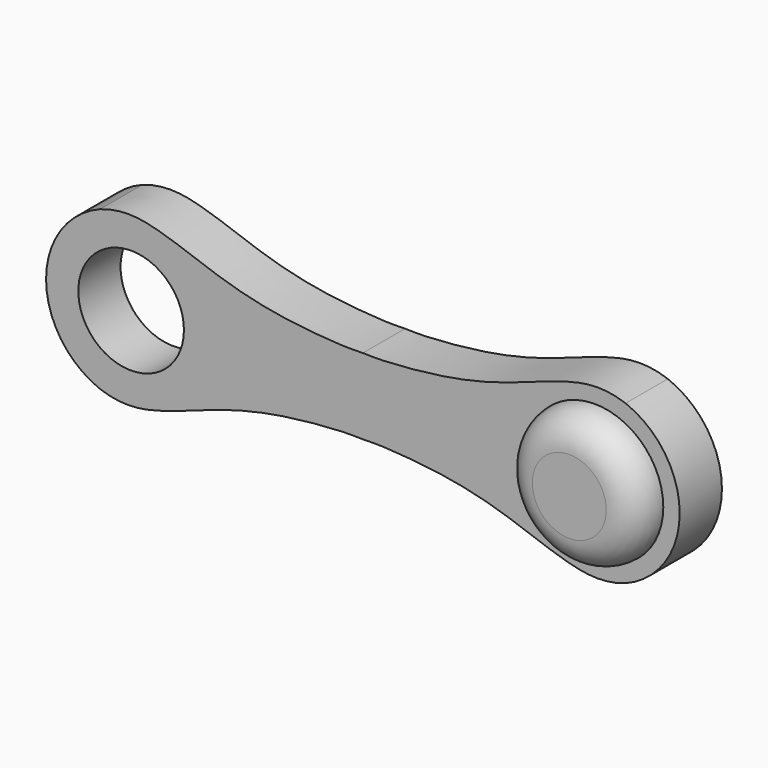
from build123d import *

# Parameters (mm, degrees)
F0_R     = 12.7
F0_R_2   = 16.51
F1_DEPTH = 12.7
F2_DEPTH = 20.32
F3_R     = 7.61999


# Not quite as in the source:
# - a fillet or chamfer is up to 0.001 mm smaller than in the source, because OpenCascade refuses the exact size


with BuildPart() as f1:
    # F0 (on Front) → F1 (new body)
    with BuildSketch(Plane.XZ):
        with BuildLine():
            add(Edge.make_bspline(
                [(63.1930127424, -19.05), (57.8929819167, -20.9148749709), (49.1822585518, -19.6780685204), (34.4123652883, -13.7010865969), (20.7204562035, -10.3509186108), (5.798157397, -8.9775289718), (1.5977957695, -9.0970061045), (0, -9.1456407681)],
                knots=[0, 0, 0, 0, 0.2119684652, 0.4335943825, 0.6511337867, 0.8674060842, 1, 1, 1, 1], degree=3))
            ThreePointArc((63.1930127424, -19.05), (76.2, 0), (63.1930127424, 19.05))
            add(Edge.make_bspline(
                [(63.1930127424, 19.05), (57.8929819167, 20.9148749709), (49.1822585518, 19.6780685204), (34.4123652883, 13.7010865969), (20.7204562035, 10.3509186108), (5.798157397, 8.9775289718), (1.5977957695, 9.0970061045), (0, 9.1456407681)],
                knots=[0, 0, 0, 0, 0.2119684652, 0.4335943825, 0.6511337867, 0.8674060842, 1, 1, 1, 1], degree=3))
            add(Edge.make_bspline(
                [(-63.1930127424, 19.05), (-57.8929819167, 20.9148749709), (-49.1822585518, 19.6780685204), (-34.4123652883, 13.7010865969), (-20.7204562035, 10.3509186108), (-5.798157397, 8.9775289718), (-1.5977957695, 9.0970061045), (0, 9.1456407681)],
                knots=[0, 0, 0, 0, 0.2119684652, 0.4335943825, 0.6511337867, 0.8674060842, 1, 1, 1, 1], degree=3))
            ThreePointArc((-63.1930127424, 19.05), (-76.2, 0), (-63.1930127424, -19.05))
            add(Edge.make_bspline(
                [(-63.1930127424, -19.05), (-57.8929819167, -20.9148749709), (-49.1822585518, -19.6780685204), (-34.4123652883, -13.7010865969), (-20.7204562035, -10.3509186108), (-5.798157397, -8.9775289718), (-1.5977957695, -9.0970061045), (0, -9.1456407681)],
                knots=[0, 0, 0, 0, 0.2119684652, 0.4335943825, 0.6511337867, 0.8674060842, 1, 1, 1, 1], degree=3))
        make_face()
        with Locations((-55.7462159306, 0)):
            Circle(F0_R, mode=Mode.SUBTRACT)
        with Locations((55.7462159306, 0)):
            Circle(F0_R_2, mode=Mode.SUBTRACT)
    extrude(amount=F1_DEPTH)

    # F0 (on Front) → F2 (join)
    with BuildSketch(Plane.XZ):
        with Locations((55.7462159306, 0)):
            Circle(F0_R_2)
    extrude(amount=F2_DEPTH)

    # F3 (radius 7.62 in the source; OpenCascade refuses exactly that, so slightly less here)
    f3_edges = [f1.edges().sort_by_distance(p)[0] for p in [
        (39.236216, -20.32, 0),
    ]]
    fillet(f3_edges, radius=F3_R)


solid = f1.part
